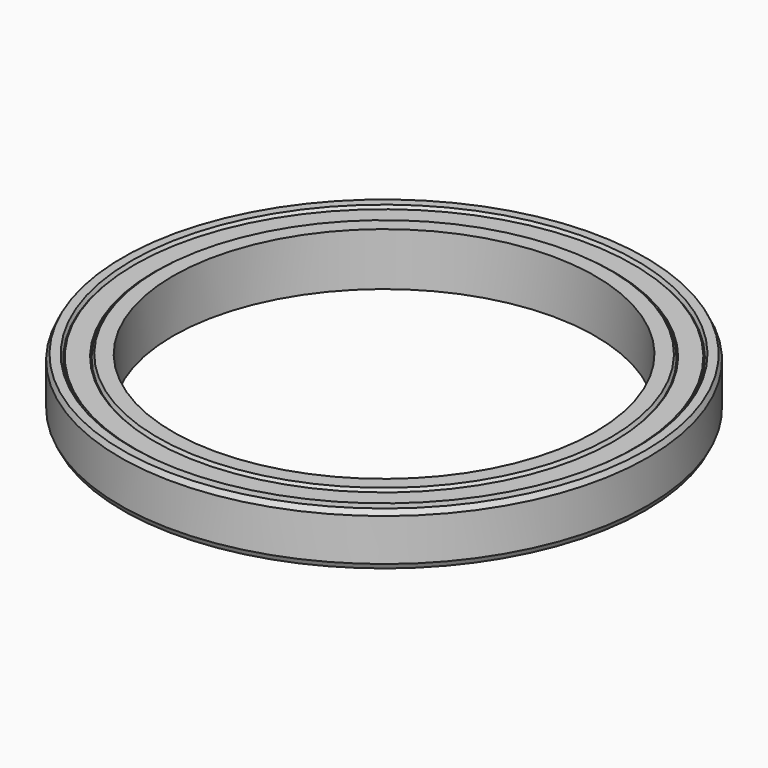
from build123d import *

# Parameters (mm, degrees)
F0_R     = 50
F0_R_2   = 40
F1_DEPTH = 10
F5_SIZE2 = 0.5
F5_SIZE  = 1


# Not quite as in the source:
# - a pattern or mirror of a feature is missing from the dataset's text; its kind, count and spacing are read off the source's solid


with BuildPart() as f1:
    # F0 (on Top) → F1 (new body)
    with BuildSketch(Plane.XY):
        Circle(F0_R)
        Circle(F0_R_2, mode=Mode.SUBTRACT)
    extrude(amount=F1_DEPTH)

    # F2 (on Front) → F3 (revolve, cut)
    with BuildSketch(Plane.XZ):
        Polygon((-50, 13.4113135189), (-50, 10), (-47.8474881957, 10), (-47.4599111567, 9.3286968768), (-47.3599111567, 9.3286968768), (-47.2283720253, 9.5565293356), (-43.498182123, 9.5565293356), (-43.3666429916, 9.3286968768), (-43.2666429916, 9.3286968768), (-42.8790659527, 10), (-40, 10), (-40, 13.4113135189), align=None)
    f3 = revolve(axis=Axis((0, 0, 10.9280112665), (0, 0, 1)), mode=Mode.SUBTRACT)

    # F3_copies: F3 across plane
    add(f3.mirror(Plane(origin=(0, 0, 5), x_dir=(-1, 0, 0), z_dir=(0, 0, -1))), mode=Mode.SUBTRACT)

    # F5
    f5_edges = [f1.edges().sort_by_distance(p)[0] for p in [
        (-50, 0, 10),
        (-50, 0, 0),
    ]]
    f5_side = f1.faces().sort_by_distance((-50, 0, 5))[0]
    chamfer(f5_edges, length=F5_SIZE, length2=F5_SIZE2, reference=f5_side)


solid = f1.part
